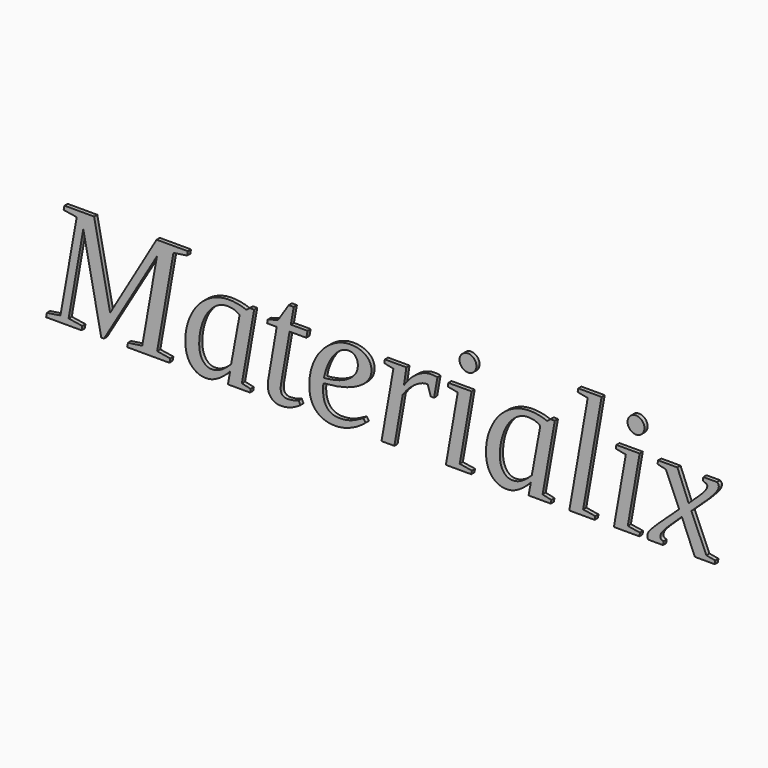
from build123d import *

# Parameters (mm, degrees)
F0_TEXT_SIZE = 80.6463546016
F1_DEPTH     = 2


# Not quite as in the source:
# - Text() gives the source's letters only with a copy of the font that has no kerning and outlines rounded to 1/6400 em; it was checked with that copy


with BuildPart() as f1:
    # F0 (on Front) → F1 (new body)
    with BuildSketch(Plane.XZ):
        with Locations((-97.2084850073, -24.7659031302)):
            Text('Materialix', F0_TEXT_SIZE, font='Tinos', font_style=FontStyle.ITALIC, text_align=(TextAlign.LEFT, TextAlign.BOTTOM))
    extrude(amount=F1_DEPTH)


solid = f1.part
